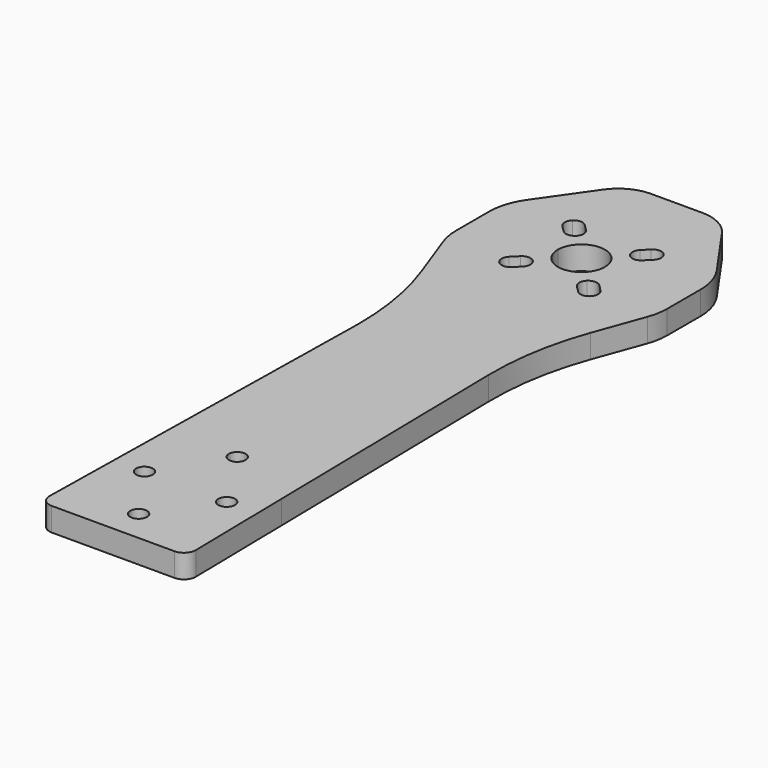
from build123d import *

# Parameters (mm, degrees)
F0_R     = 1.425
F1_DEPTH = 4


# Not quite as in the source:
# - a feature names something its author has since deleted; it is built from what else it names


with BuildPart() as f1:
    # F0 (on Top) → F1 (new body)
    with BuildSketch(Plane.XY):
        with BuildLine():
            ThreePointArc((-32.6695806955, 2.2650205107), (-31.9914759382, 11.3900208154), (-29.6618269361, 20.2386473839))
            Line((-29.6618269361, 20.2386473839), (-32.8313113004, 11.5305606615))
            Line((-32.8313113004, 11.5305606615), (-32.6695806955, 2.2650205107))
        make_face()
        with BuildLine():
            Line((-55.2126988023, 11.5305606615), (-58.3821831004, 20.2386472017))
            ThreePointArc((-58.3821831004, 20.2386472017), (-56.126426517, 11.8200489678), (-55.3668141772, 3.1376401385))
            ThreePointArc((-55.3668141772, 3.1376401385), (-55.3687180209, 2.7013137107), (-55.3744294072, 2.2650205107))
            Line((-55.3744294072, 2.2650205107), (-55.2126988023, 11.5305606615))
        make_face()
        with BuildLine():
            Line((-39.6659744052, 56.5204558903), (-48.3780356975, 56.5204558903))
            ThreePointArc((-48.3780356975, 56.5204558903), (-51.6102759902, 55.7295317226), (-54.1121000075, 53.5354909448))
            Line((-54.1121000075, 53.5354909448), (-60.2135254943, 44.8217522976))
            ThreePointArc((-60.2135254943, 44.8217522976), (-61.5591745589, 42.0930459292), (-62.0220050514, 39.0859879341))
            Line((-62.0220050514, 39.0859879341), (-62.0220050514, 36.2389758229))
            Line((-62.0220050514, 36.2389758229), (-48.0220050514, 36.2389758229))
            ThreePointArc((-48.0220050514, 36.2389758229), (-44.0220050514, 40.2389758229), (-40.0220050514, 36.2389758229))
            Line((-40.0220050514, 36.2389758229), (-26.0220050514, 36.2389758229))
            Line((-26.0220050514, 36.2389758229), (-26.0220050514, 39.0859879341))
            ThreePointArc((-26.0220050514, 39.0859879341), (-26.4848355439, 42.0930459292), (-27.8304846085, 44.8217522976))
            Line((-27.8304846085, 44.8217522976), (-33.9319100952, 53.5354909448))
            ThreePointArc((-33.9319100952, 53.5354909448), (-36.4337341126, 55.7295317226), (-39.6659744052, 56.5204558903))
        make_face()
        with BuildLine():
            Line((-49.6788593009, 44.017150416), (-48.6181991291, 42.9564902442))
            ThreePointArc((-48.6181991291, 42.9564902442), (-48.1788593009, 41.8958300724), (-48.6181991291, 40.8351699006))
            ThreePointArc((-48.6181991291, 40.8351699006), (-49.6788593009, 40.3958300724), (-50.7395194726, 40.8351699006))
            Line((-50.7395194726, 40.8351699006), (-51.8001796444, 41.8958300724))
            ThreePointArc((-51.8001796444, 41.8958300724), (-52.2395194726, 42.9564902442), (-51.8001796444, 44.017150416))
            ThreePointArc((-51.8001796444, 44.017150416), (-50.7395194726, 44.4564902442), (-49.6788593009, 44.017150416))
        make_face(mode=Mode.SUBTRACT)
        with BuildLine():
            ThreePointArc((-36.2438304583, 44.017150416), (-35.8044906301, 42.9564902442), (-36.2438304583, 41.8958300724))
            Line((-36.2438304583, 41.8958300724), (-37.3044906301, 40.8351699006))
            ThreePointArc((-37.3044906301, 40.8351699006), (-38.3651508019, 40.3958300724), (-39.4258109737, 40.8351699006))
            ThreePointArc((-39.4258109737, 40.8351699006), (-39.8651508019, 41.8958300724), (-39.4258109737, 42.9564902442))
            Line((-39.4258109737, 42.9564902442), (-38.3651508019, 44.017150416))
            ThreePointArc((-38.3651508019, 44.017150416), (-37.3044906301, 44.4564902442), (-36.2438304583, 44.017150416))
        make_face(mode=Mode.SUBTRACT)
        with BuildLine():
            Line((-31.557524447, -61.4446392968), (-31.8823640322, -42.8345919221))
            ThreePointArc((-31.8823640322, -42.8345919221), (-44.0220050514, -43.7610241771), (-56.1616460705, -42.8345919221))
            Line((-56.1616460705, -42.8345919221), (-56.4864856557, -61.4446392968))
            ThreePointArc((-56.4864856557, -61.4446392968), (-55.9132911637, -62.8813626383), (-54.4867902654, -63.4795441097))
            Line((-54.4867902654, -63.4795441097), (-33.5572198373, -63.4795441097))
            ThreePointArc((-33.5572198373, -63.4795441097), (-32.130718939, -62.8813626383), (-31.557524447, -61.4446392968))
        make_face()
        with Locations((-51.0220050514, -58.0545441097)):
            Circle(F0_R, mode=Mode.SUBTRACT)
        with Locations((-51.0220050514, -48.0545441097)):
            Circle(F0_R, mode=Mode.SUBTRACT)
        with Locations((-44.0220050514, -58.0545441097)):
            Circle(F0_R, mode=Mode.SUBTRACT)
        with Locations((-37.0220050514, -58.0545441097)):
            Circle(F0_R, mode=Mode.SUBTRACT)
        with Locations((-37.0220050514, -48.0545441097)):
            Circle(F0_R, mode=Mode.SUBTRACT)
        with BuildLine():
            Line((-48.0220050514, 36.2389758229), (-62.0220050514, 36.2389758229))
            Line((-62.0220050514, 36.2389758229), (-62.0220050514, 32.00224563))
            ThreePointArc((-62.0220050514, 32.00224563), (-61.8700825815, 30.2657638533), (-61.4189312592, 28.5820441968))
            Line((-61.4189312592, 28.5820441968), (-58.3821831004, 20.2386472017))
            Line((-58.3821831004, 20.2386472017), (-55.2126988023, 11.5305606615))
            Line((-55.2126988023, 11.5305606615), (-55.3744294072, 2.2650205107))
            Line((-55.3744294072, 2.2650205107), (-56.1616460705, -42.8345919221))
            ThreePointArc((-56.1616460705, -42.8345919221), (-44.0220050514, -43.7610241771), (-31.8823640322, -42.8345919221))
            Line((-31.8823640322, -42.8345919221), (-32.6695806955, 2.2650205107))
            Line((-32.6695806955, 2.2650205107), (-32.8313113004, 11.5305606615))
            Line((-32.8313113004, 11.5305606615), (-29.6618269361, 20.2386473839))
            Line((-29.6618269361, 20.2386473839), (-26.6250788435, 28.5820441968))
            ThreePointArc((-26.6250788435, 28.5820441968), (-26.1739275213, 30.2657638533), (-26.0220050514, 32.00224563))
            Line((-26.0220050514, 32.00224563), (-26.0220050514, 36.2389758229))
            Line((-26.0220050514, 36.2389758229), (-40.0220050514, 36.2389758229))
            ThreePointArc((-40.0220050514, 36.2389758229), (-40.3264869213, 34.7082420935), (-41.1935779266, 33.4105486982))
            ThreePointArc((-41.1935779266, 33.4105486982), (-44.0220050514, 32.2389758229), (-46.8504321761, 33.4105486982))
            ThreePointArc((-46.8504321761, 33.4105486982), (-47.7175231814, 34.7082420935), (-48.0220050514, 36.2389758229))
        make_face()
        with Locations((-44.0220050514, -37.0545441097)):
            Circle(F0_R, mode=Mode.SUBTRACT)
        with BuildLine():
            ThreePointArc((-50.7395194726, 31.6427817452), (-49.6788593009, 32.0821215734), (-48.6181991291, 31.6427817452))
            ThreePointArc((-48.6181991291, 31.6427817452), (-48.1788593009, 30.5821215734), (-48.6181991291, 29.5214614017))
            Line((-48.6181991291, 29.5214614017), (-49.6788593009, 28.4608012299))
            ThreePointArc((-49.6788593009, 28.4608012299), (-50.7395194726, 28.0214614017), (-51.8001796444, 28.4608012299))
            ThreePointArc((-51.8001796444, 28.4608012299), (-52.2395194726, 29.5214614017), (-51.8001796444, 30.5821215734))
            Line((-51.8001796444, 30.5821215734), (-50.7395194726, 31.6427817452))
        make_face(mode=Mode.SUBTRACT)
        with BuildLine():
            ThreePointArc((-39.4258109737, 29.5214614017), (-39.8651508019, 30.5821215734), (-39.4258109737, 31.6427817452))
            ThreePointArc((-39.4258109737, 31.6427817452), (-38.3651508019, 32.0821215734), (-37.3044906301, 31.6427817452))
            Line((-37.3044906301, 31.6427817452), (-36.2438304583, 30.5821215734))
            ThreePointArc((-36.2438304583, 30.5821215734), (-35.8044906301, 29.5214614017), (-36.2438304583, 28.4608012299))
            ThreePointArc((-36.2438304583, 28.4608012299), (-37.3044906301, 28.0214614017), (-38.3651508019, 28.4608012299))
            Line((-38.3651508019, 28.4608012299), (-39.4258109737, 29.5214614017))
        make_face(mode=Mode.SUBTRACT)
        with Locations((-51.0220050514, -58.0545441097)):
            Circle(F0_R)
        with Locations((-37.0220050514, -58.0545441097)):
            Circle(F0_R)
    extrude(amount=F1_DEPTH)


solid = f1.part
